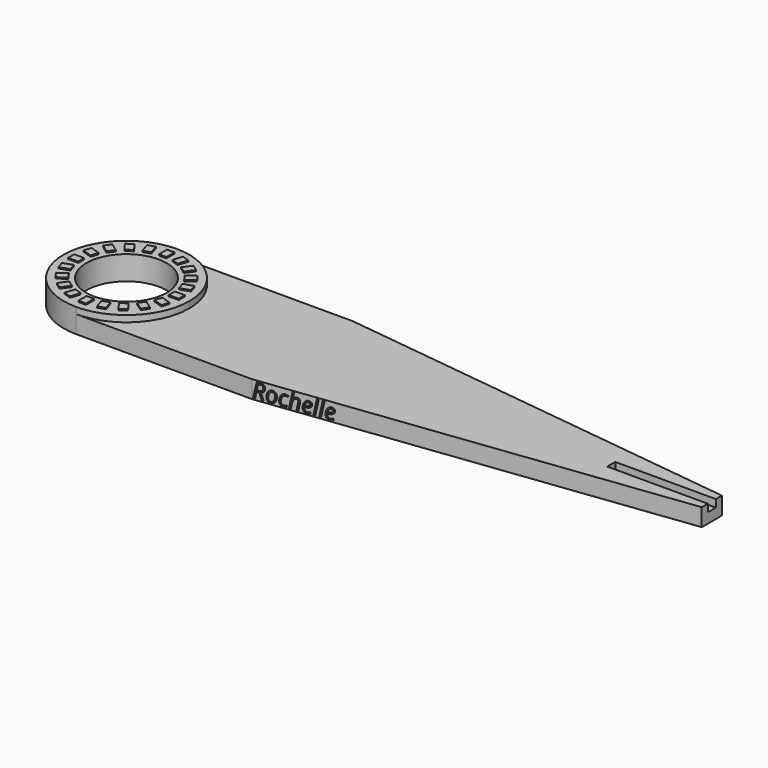
from build123d import *

# Parameters (mm, degrees)
F0_R         = 8
F1_DEPTH     = 3.5
F2_R         = 8
F3_DEPTH     = 1.27
F4_W         = 1.5
F4_H         = 2
F4_W_2       = 2
F4_H_2       = 1.5
F5_DEPTH     = 0.25
F6_W         = 20
F6_H         = 2
F7_DEPTH     = 1.5
F8_TEXT_SIZE = 4.1666666667
F9_DEPTH     = 0.3


# Not quite as in the source:
# - Text() gives the source's letters only with a copy of the font that has no kerning and outlines rounded to 1/6400 em; it was checked with that copy


with BuildPart() as f1:
    # F0 (on Top) → F1 (new body)
    with BuildSketch(Plane.XY):
        with BuildLine():
            ThreePointArc((0, -12.5), (8.8388347648, -8.8388347648), (12.5, 0))
            ThreePointArc((12.5, 0), (8.8388347648, 8.8388347648), (0, 12.5))
            ThreePointArc((0, 12.5), (-12.5, 0), (0, -12.5))
        make_face()
        Circle(F0_R, mode=Mode.SUBTRACT)
        with BuildLine():
            ThreePointArc((0, 12.5), (8.8388347648, 8.8388347648), (12.5, 0))
            ThreePointArc((12.5, 0), (8.8388347648, -8.8388347648), (0, -12.5))
            Line((0, -12.5), (35, -12.5))
            Line((35, -12.5), (116.3887844346, -2.5067138408))
            Line((116.3887844346, -2.5067138408), (116.3887844346, 2.5067138408))
            Line((116.3887844346, 2.5067138408), (35, 12.5))
            Line((35, 12.5), (0, 12.5))
        make_face()
    extrude(amount=F1_DEPTH)

    # F2 (on face) → F3 (join)
    with BuildSketch(Plane.XY.offset(3.5)):
        with BuildLine():
            ThreePointArc((0, -12.5), (8.8388347648, -8.8388347648), (12.5, 0))
            ThreePointArc((12.5, 0), (8.8388347648, 8.8388347648), (0, 12.5))
            ThreePointArc((0, 12.5), (-12.5, 0), (0, -12.5))
        make_face()
        Circle(F2_R, mode=Mode.SUBTRACT)
    extrude(amount=F3_DEPTH)

    # F4 (on face) → F5 (join)
    with BuildSketch(Plane.XY.offset(4.77)):
        with Locations((0, 10)):
            Rectangle(F4_W, F4_H)
        Polygon((-2.0678605622, 8.7912713924), (-2.6858945509, 10.693384425), (-4.1124793253, 10.2298589335), (-3.4944453366, 8.3277459009), align=None)
        Polygon((-4.6833045249, 7.7219918886), (-5.8588750294, 9.3400258773), (-7.072400521, 8.4583479989), (-5.8968300164, 6.8403140102), align=None)
        Polygon((-6.8403140102, 5.8968300164), (-8.4583479989, 7.072400521), (-9.3400258773, 5.8588750294), (-7.7219918886, 4.6833045249), align=None)
        Polygon((-8.3277459009, 3.4944453366), (-10.2298589335, 4.1124793253), (-10.693384425, 2.6858945509), (-8.7912713924, 2.0678605622), align=None)
        with Locations((-10, 0)):
            Rectangle(F4_W_2, F4_H_2)
        Polygon((-8.7912713924, -2.0678605622), (-10.693384425, -2.6858945509), (-10.2298589335, -4.1124793253), (-8.3277459009, -3.4944453366), align=None)
        Polygon((-7.7219918886, -4.6833045249), (-9.3400258773, -5.8588750294), (-8.4583479989, -7.072400521), (-6.8403140102, -5.8968300164), align=None)
        Polygon((-5.8968300164, -6.8403140102), (-7.072400521, -8.4583479989), (-5.8588750294, -9.3400258773), (-4.6833045249, -7.7219918886), align=None)
        Polygon((-3.4944453366, -8.3277459009), (-4.1124793253, -10.2298589335), (-2.6858945509, -10.693384425), (-2.0678605622, -8.7912713924), align=None)
        with Locations((0, -10)):
            Rectangle(F4_W, F4_H)
        Polygon((2.0678605622, -8.7912713924), (2.6858945509, -10.693384425), (4.1124793253, -10.2298589335), (3.4944453366, -8.3277459009), align=None)
        Polygon((4.6833045249, -7.7219918886), (5.8588750294, -9.3400258773), (7.072400521, -8.4583479989), (5.8968300164, -6.8403140102), align=None)
        Polygon((6.8403140102, -5.8968300164), (8.4583479989, -7.072400521), (9.3400258773, -5.8588750294), (7.7219918886, -4.6833045249), align=None)
        Polygon((8.3277459009, -3.4944453366), (10.2298589335, -4.1124793253), (10.693384425, -2.6858945509), (8.7912713924, -2.0678605622), align=None)
        with Locations((10, 0)):
            Rectangle(F4_W_2, F4_H_2)
        Polygon((8.7912713924, 2.0678605622), (10.693384425, 2.6858945509), (10.2298589335, 4.1124793253), (8.3277459009, 3.4944453366), align=None)
        Polygon((7.7219918886, 4.6833045249), (9.3400258773, 5.8588750294), (8.4583479989, 7.072400521), (6.8403140102, 5.8968300164), align=None)
        Polygon((5.8968300164, 6.8403140102), (7.072400521, 8.4583479989), (5.8588750294, 9.3400258773), (4.6833045249, 7.7219918886), align=None)
        Polygon((3.4944453366, 8.3277459009), (4.1124793253, 10.2298589335), (2.6858945509, 10.693384425), (2.0678605622, 8.7912713924), align=None)
    extrude(amount=F5_DEPTH)

    # F6 (on face) → F7 (cut)
    with BuildSketch(Plane.XY.offset(3.5)):
        with Locations((106.3887844346, 0)):
            Rectangle(F6_W, F6_H)
    extrude(amount=-F7_DEPTH, mode=Mode.SUBTRACT)

    # F8 (on face) → F9 (cut)
    with BuildSketch(Plane(origin=(2.0318366377, -16.5479814622, 0), x_dir=(0.9925461516, 0.1218693434, 0), z_dir=(0.1218693434, -0.9925461516, 0))):
        with Locations((33.2157485149, 0.25)):
            Text('Rochelle', F8_TEXT_SIZE, font='Open Sans', font_style=FontStyle.ITALIC, text_align=(TextAlign.LEFT, TextAlign.BOTTOM))
    extrude(amount=-F9_DEPTH, mode=Mode.SUBTRACT)


solid = f1.part
